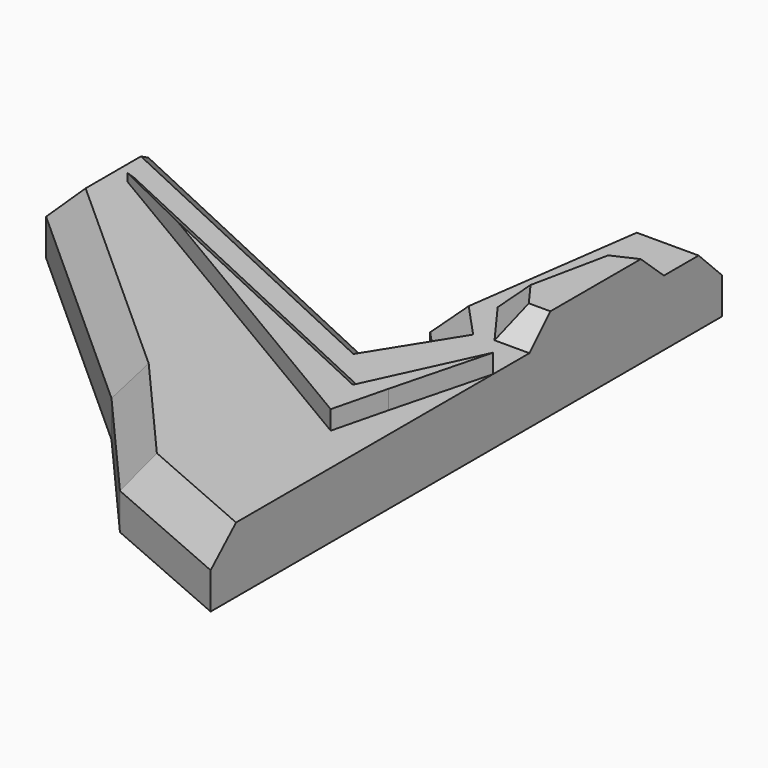
from build123d import *

# Parameters (mm, degrees)
F1_DEPTH     = 11.43
F2_SIZE      = 5.08
F4_DEPTH     = 4.572
F5_T4_DEPTH  = 35.6101050897
F5_T9_DEPTH  = 44.6545724626
F5_T14_DEPTH = 36.379020654
F5_T19_DEPTH = 32.4730482843
F7_DEPTH     = 3.302
F8_T4_DEPTH  = 87.5344337201


# Not quite as in the source:
# - a fillet or chamfer that OpenCascade refuses, or shapes differently, is made with other operations: its cross-section is extruded or revolved along the edge and cut away or added


with BuildPart() as f1:
    # F0 (on Top) → F1 (new body)
    with BuildSketch(Plane.XY):
        Polygon((0, -46.853557229), (0, 64.6125674248), (-15.2085125446, 64.6125674248), (-20.4984303564, 26.6385115683), (-15.7752875239, 21.5375181288), (-20.4984303564, 13.9804948121), (-82.6549530029, 42.8861156106), (-82.6549530029, 20.5928906798), (-42.2248728573, -15.6808290631), (-24.276940152, -36.2737216055), align=None)
    extrude(amount=F1_DEPTH)

    # F2
    f2_edges = [f1.edges().sort_by_distance(p)[0] for p in [
        (-51.576692, 28.433305, 11.43),
        (-82.654953, 31.739503, 11.43),
        (-62.439913, 2.456031, 11.43),
        (-18.136859, 17.759006, 11.43),
        (-18.136859, 24.088015, 11.43),
        (-17.853471, 45.625539, 11.43),
        (-7.604256, 64.612567, 11.43),
        (-33.250907, -25.977275, 11.43),
        (-12.13847, -41.563639, 11.43),
    ]]
    chamfer(f2_edges, length=F2_SIZE)

    # F3 (on face) → F4 (join)
    with BuildSketch(Plane.XY.offset(11.43)):
        Polygon((0, 22.1388745617), (0, 52.5213219225), (-8.6118569598, 48.5538840294), (-12.3903686181, 30.4170250893), (-6.3447491266, 22.1388745617), align=None)
    extrude(amount=F4_DEPTH)

    # F5: chamfer of 5.08 on 4 edges, made by hand


with BuildPart() as f5_tool2:
    # F5_s3 → F5_t4 (new body)
    with BuildSketch(Plane(origin=(31.8255199814, 14.6618522037, 0), x_dir=(0, 0, 1), z_dir=(-0.9082507089, -0.418426397, 0))):
        Polygon((10.922, 47.7025278707), (16.002, 42.6225278707), (16.002, 47.7025278707), align=None)
    extrude(amount=F5_T4_DEPTH)

    split(bisect_by=Plane.XY.offset(11.43), keep=Keep.TOP)


with BuildPart() as f1_1:
    add(f1.part)

    # F5_t1: cut F5_tool2
    add(f5_tool2.part, mode=Mode.SUBTRACT)


with BuildPart() as f5_tool7:
    # F5_s8 → F5_t9 (new body)
    with BuildSketch(Plane(origin=(12.0008759003, 57.6042137868, 0), x_dir=(0, 0, 1), z_dir=(-0.203954222, -0.9789804264, 0))):
        Polygon((10.922, 18.3336090407), (16.002, 13.2536090407), (16.002, 18.3336090407), align=None)
    extrude(amount=F5_T9_DEPTH)

    split(bisect_by=Plane.XY.offset(11.43), keep=Keep.TOP)


with BuildPart() as f1_2:
    add(f1_1.part)

    # F5_t6: cut F5_tool7
    add(f5_tool7.part, mode=Mode.SUBTRACT)


with BuildPart() as f5_tool12:
    # F5_s13 → F5_t14 (new body)
    with BuildSketch(Plane(origin=(-26.5018256682, 36.2884403239, 0), x_dir=(0, 0, 1), z_dir=(0.5897750216, -0.8075675971, 0))):
        Polygon((10.922, -7.9331414154), (16.002, -13.0131414154), (16.002, -7.9331414154), align=None)
    extrude(amount=F5_T14_DEPTH)

    split(bisect_by=Plane.XY.offset(11.43), keep=Keep.TOP)


with BuildPart() as f1_3:
    add(f1_2.part)

    # F5_t11: cut F5_tool12
    add(f5_tool12.part, mode=Mode.SUBTRACT)


with BuildPart() as f5_tool17:
    # F5_s18 → F5_t19 (new body)
    with BuildSketch(Plane.YZ.offset(-19.4088987055)):
        Polygon((22.1388745617, 10.922), (27.2188745617, 16.002), (22.1388745617, 16.002), align=None)
    extrude(amount=F5_T19_DEPTH)

    split(bisect_by=Plane.XY.offset(11.43), keep=Keep.TOP)


with BuildPart() as f1_4:
    add(f1_3.part)

    # F5_t16: cut F5_tool17
    add(f5_tool17.part, mode=Mode.SUBTRACT)

    # F6 (on face) → F7 (join)
    with BuildSketch(Plane.XY.offset(11.43)):
        Polygon((-4.4554928318, -2.4560331367), (0, 14.7361988202), (-6.8530052353, 0), (-74.3786075584, 31.4024879744), (-74.3786075584, 27.9609914869), (-6.8530052353, -12.1079402775), align=None)
    extrude(amount=F7_DEPTH)

    # F8: chamfer of 5.08 on 1 edges, made by hand


with BuildPart() as f8_tool2:
    # F8_s3 → F8_t4 (new body)
    with BuildSketch(Plane(origin=(-5.6344557861, 2.6202791827, 0), x_dir=(0, 0, 1), z_dir=(-0.9067455979, 0.4216781007, 0))):
        Polygon((9.652, -2.8897622316), (14.732, -7.9697622316), (14.732, -2.8897622316), align=None)
    extrude(amount=F8_T4_DEPTH)

    split(bisect_by=Plane.XY.offset(11.43), keep=Keep.TOP)


with BuildPart() as f1_5:
    add(f1_4.part)

    # F8_t1: cut F8_tool2
    add(f8_tool2.part, mode=Mode.SUBTRACT)


solid = f1_5.part
